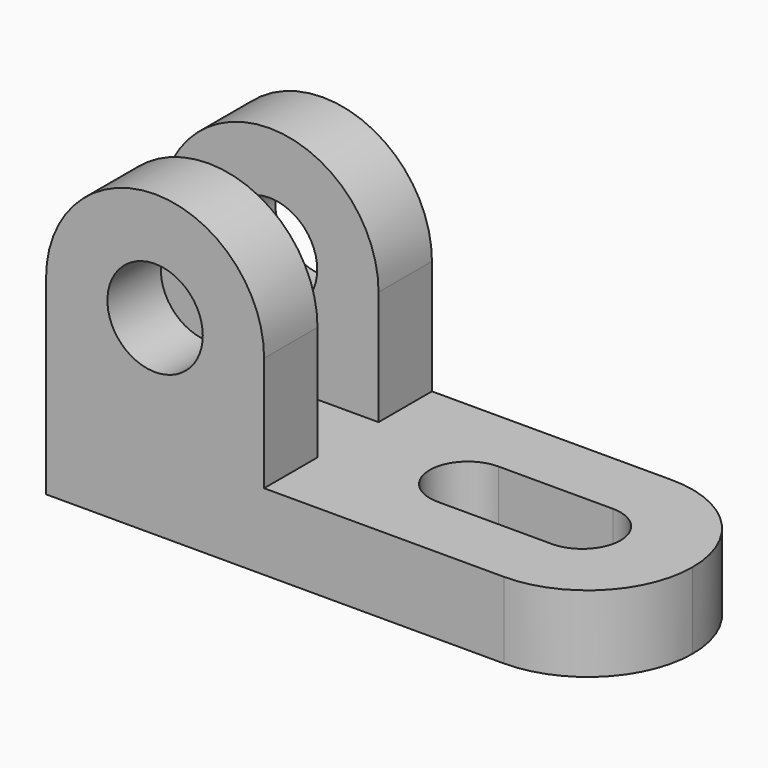
from build123d import *

# Parameters (mm, degrees)
F0_R          = 10
F1_DEPTH      = 22
F1_DEPTH_BACK = 22
F2_DEPTH      = 8
F2_DEPTH_BACK = 8
F3_R          = 21.99999
F5_DEPTH      = 25


# Not quite as in the source:
# - a fillet or chamfer is up to 0.001 mm smaller than in the source, because OpenCascade refuses the exact size


with BuildPart() as f1:
    # F0 (on Front) → F1 (new body, two sides)
    with BuildSketch(Plane.XZ) as f1_sk:
        with BuildLine():
            Line((0, 40), (0, 16))
            Line((0, 16), (45.7235909998, 16))
            Line((45.7235909998, 16), (45.7235909998, 40))
            ThreePointArc((45.7235909998, 40), (22.8617954999, 62.8617954999), (0, 40))
        make_face()
        with Locations((22.8617954999, 40)):
            Circle(F0_R, mode=Mode.SUBTRACT)
        Polygon((0, 16), (0, 0), (118, 0), (118, 16), (45.7235909998, 16), align=None)
    extrude(amount=F1_DEPTH)
    extrude(f1_sk.sketch, amount=-F1_DEPTH_BACK)

    # F0 (on Front) → F2 (cut, two sides)
    with BuildSketch(Plane.XZ) as f2_sk:
        with BuildLine():
            Line((45.7235909998, 16), (118, 16))
            Line((118, 16), (118, 71.8919485807))
            Line((118, 71.8919485807), (0, 71.8919485807))
            Line((0, 71.8919485807), (0, 40))
            ThreePointArc((0, 40), (22.8617954999, 62.8617954999), (45.7235909998, 40))
            Line((45.7235909998, 40), (45.7235909998, 16))
        make_face()
        with BuildLine():
            Line((0, 40), (0, 16))
            Line((0, 16), (45.7235909998, 16))
            Line((45.7235909998, 16), (45.7235909998, 40))
            ThreePointArc((45.7235909998, 40), (22.8617954999, 62.8617954999), (0, 40))
        make_face()
        with Locations((22.8617954999, 40)):
            Circle(F0_R, mode=Mode.SUBTRACT)
    extrude(amount=-F2_DEPTH, mode=Mode.SUBTRACT)
    extrude(f2_sk.sketch, amount=F2_DEPTH_BACK, mode=Mode.SUBTRACT)

    # F3 (radius 22 in the source; OpenCascade refuses exactly that, so slightly less here)
    f3_edges = [f1.edges().sort_by_distance(p)[0] for p in [
        (118, -22, 8),
        (118, 22, 8),
    ]]
    fillet(f3_edges, radius=F3_R)

    # F4 (on face) → F5 (cut)
    with BuildSketch(Plane.XY.offset(16)):
        with BuildLine():
            ThreePointArc((70.8617954999, 8), (62.8617954999, 0), (70.8617954999, -8))
            Line((70.8617954999, -8), (94.8617954999, -8))
            ThreePointArc((94.8617954999, -8), (102.8617954999, 0), (94.8617954999, 8))
            Line((94.8617954999, 8), (70.8617954999, 8))
        make_face()
    extrude(amount=-F5_DEPTH, mode=Mode.SUBTRACT)


solid = f1.part
